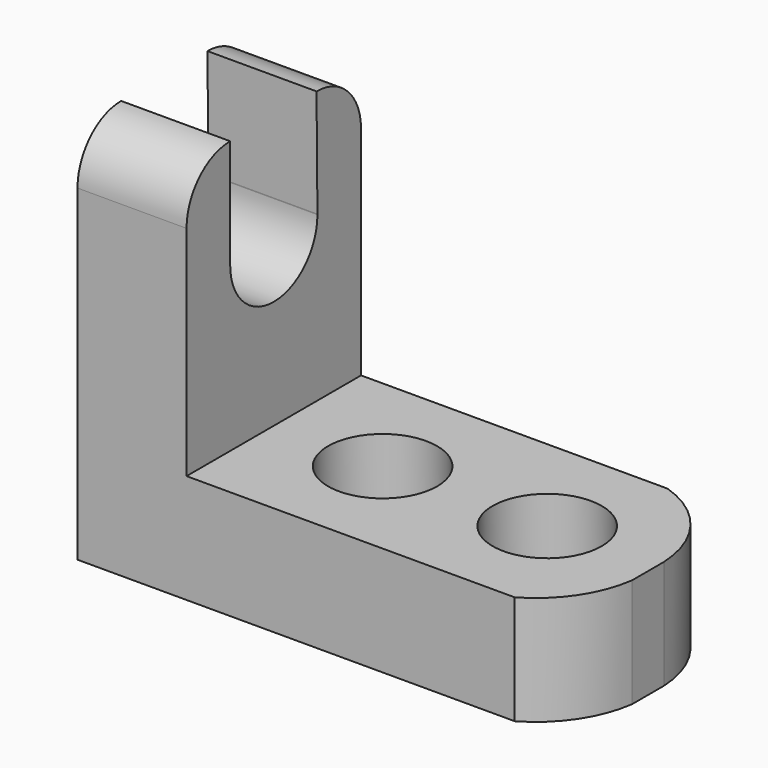
from build123d import *

# Parameters (mm, degrees)
F1_DEPTH = 25.4
F3_DEPTH = 12.7
F4_R     = 6.35
F5_DEPTH = 25.4


# Not quite as in the source:
# - ends of sketch curves that miss each other by under 0.0002 mm in the source are joined


with BuildPart() as f1:
    # F0 (on Front) → F1 (new body)
    with BuildSketch(Plane.XZ):
        Polygon((0, 44.45), (0, 0), (57.15, 0), (57.15, 12.7), (12.7, 12.7), (12.7, 44.45), align=None)
    extrude(amount=F1_DEPTH)

    # F2 (on face) → F3 (cut)
    with BuildSketch(Plane.YZ.offset(12.7)):
        with BuildLine():
            Line((-12.7, 31.75), (-19.05, 31.75))
            ThreePointArc((-19.05, 31.75), (-12.7, 25.4), (-6.35, 31.75))
            Line((-6.35, 31.75), (-12.7, 31.75))
        make_face()
        with BuildLine():
            Line((-19.05, 44.45), (-19.05, 31.75))
            ThreePointArc((-19.05, 31.75), (-12.732894977, 38.0999147963), (-6.3503408124, 31.8157890712))
            Line((-6.3503408124, 31.8157890712), (-6.4812591328, 44.45))
            Line((-6.4812591328, 44.45), (-19.05, 44.45))
        make_face()
        with BuildLine():
            ThreePointArc((-6.3503408124, 31.8157890712), (-12.732894977, 38.0999147963), (-19.05, 31.75))
            Line((-19.05, 31.75), (-12.7, 31.75))
            Line((-12.7, 31.75), (-6.35, 31.75))
            ThreePointArc((-6.35, 31.75), (-6.3500852037, 31.782894977), (-6.3503408124, 31.8157890712))
        make_face()
        with BuildLine():
            ThreePointArc((-25.4, 38.1), (-23.5401280605, 42.5901280605), (-19.05, 44.45))
            Line((-19.05, 44.45), (-25.4, 44.45))
            Line((-25.4, 44.45), (-25.4, 38.1))
        make_face()
        with BuildLine():
            Line((0, 44.45), (-6.4812591328, 44.45))
            ThreePointArc((-6.4812591328, 44.45), (-1.9444866031, 42.597935184), (0, 38.1))
            Line((0, 38.1), (0, 44.45))
        make_face()
    extrude(amount=-F3_DEPTH, mode=Mode.SUBTRACT)

    # F4 (on face) → F5 (cut)
    with BuildSketch(Plane.XY.offset(12.7)):
        with Locations((25.4, -12.7384394317)):
            Circle(F4_R)
        with Locations((44.45, -12.5940097496)):
            Circle(F4_R)
        with BuildLine():
            ThreePointArc((48.39091748, 0), (54.5541990648, -4.3642287783), (57.15, -11.4560797516))
            Line((57.15, -11.4560797516), (57.15, 0))
            Line((57.15, 0), (48.39091748, 0))
        make_face()
        with BuildLine():
            Line((57.15, -25.4), (57.15, -16.1034604334))
            ThreePointArc((57.15, -16.1034604334), (55.1119721944, -21.4757258052), (50.91496557, -25.4))
            Line((50.91496557, -25.4), (57.15, -25.4))
        make_face()
    extrude(amount=-F5_DEPTH, mode=Mode.SUBTRACT)


solid = f1.part
